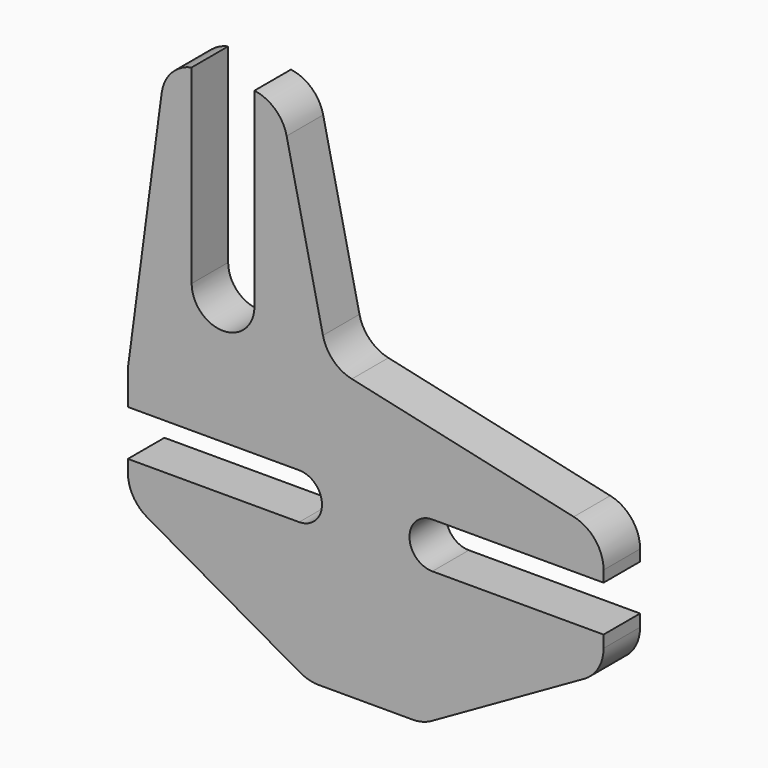
from build123d import *

# Parameters (mm, degrees)
F1_DEPTH     = 12
F2_T1_DEPTH  = 12
F2_T3_DEPTH  = 54.7223945877
F2_T5_DEPTH  = 15.3186487605
F2_T7_DEPTH  = 41.0920435526
F2_T9_DEPTH  = 25.2174840277
F2_T11_DEPTH = 25.2174840277
F2_T13_DEPTH = 41.0920435526
F2_T15_DEPTH = 52.1292425836
F2_T17_DEPTH = 51.6983242764


# Not quite as in the source:
# - a fillet or chamfer that OpenCascade refuses, or shapes differently, is made with other operations: its cross-section is extruded or revolved along the edge and cut away or added


with BuildPart() as f1:
    # F0 (on Front) → F1 (new body)
    with BuildSketch(Plane.XZ):
        with BuildLine():
            Line((-52.5, 90), (-62.5, 15))
            Line((-62.5, 15), (-62.5, 6))
            Line((-62.5, 6), (-17.5, 6))
            ThreePointArc((-17.5, 6), (-11.5, 0), (-17.5, -6))
            Line((-17.5, -6), (-62.5, -6))
            Line((-62.5, -6), (-62.5, -15))
            Line((-62.5, -15), (-15, -42))
            Line((-15, -42), (15, -42))
            Line((15, -42), (62.5, -15))
            Line((62.5, -15), (62.5, -6))
            Line((62.5, -6), (17.5, -6))
            ThreePointArc((17.5, -6), (11.5, 0), (17.5, 6))
            Line((17.5, 6), (62.5, 6))
            Line((62.5, 6), (62.5, 16.9622953511))
            Line((62.5, 16.9622953511), (-9.86454105, 33.0051278665))
            Line((-9.86454105, 33.0051278665), (-22.5, 90))
            Line((-22.5, 90), (-29.25, 90))
            Line((-29.25, 90), (-29.25, 40))
            ThreePointArc((-29.25, 40), (-37.5, 31.75), (-45.75, 40))
            Line((-45.75, 40), (-45.75, 90))
            Line((-45.75, 90), (-52.5, 90))
        make_face()
    extrude(amount=F1_DEPTH)

    # F2: fillet of radius 10 on 9 edges, made by hand

    # F2_s2 → F2_t1 (join)
    with BuildSketch(Plane.XZ):
        with BuildLine():
            ThreePointArc((-3.6448495312, 31.6262554535), (-8.5515212037, 34.3181477128), (-11.243413463, 39.2248193853))
            Line((-11.243413463, 39.2248193853), (-9.86454105, 33.0051278665))
            Line((-9.86454105, 33.0051278665), (-3.6448495312, 31.6262554535))
        make_face()
    extrude(amount=F2_T1_DEPTH)

    # F2_s4 → F2_t3 (cut)
    with BuildSketch(Plane.XZ.offset(-21.3611972939)):
        with BuildLine():
            ThreePointArc((-53.62927012, 81.5304741001), (-51.0385819893, 87.0201735553), (-45.75, 90))
            Line((-45.75, 90), (-52.5, 90))
            Line((-52.5, 90), (-53.62927012, 81.5304741001))
        make_face()
    extrude(amount=F2_T3_DEPTH, mode=Mode.SUBTRACT)

    # F2_s6 → F2_t5 (cut)
    with BuildSketch(Plane.XZ.offset(-1.6593243803)):
        with BuildLine():
            ThreePointArc((-62.4122790068, 15.6579074488), (-62.478045652, 14.9985428246), (-62.5, 14.3362702479))
            Line((-62.5, 14.3362702479), (-62.5, 15))
            Line((-62.5, 15), (-62.4122790068, 15.6579074488))
        make_face()
    extrude(amount=F2_T5_DEPTH, mode=Mode.SUBTRACT)

    # F2_s8 → F2_t7 (cut)
    with BuildSketch(Plane.XZ.offset(-14.5460217763)):
        with BuildLine():
            ThreePointArc((-57.4416662495, -17.875263395), (-61.1433981308, -14.2106735867), (-62.5, -9.1815912895))
            Line((-62.5, -9.1815912895), (-62.5, -15))
            Line((-62.5, -15), (-57.4416662495, -17.875263395))
        make_face()
    extrude(amount=F2_T7_DEPTH, mode=Mode.SUBTRACT)

    # F2_s10 → F2_t9 (cut)
    with BuildSketch(Plane.XZ.offset(-6.6087420138)):
        with BuildLine():
            ThreePointArc((-12.3565031945, -42), (-14.9122104297, -41.6679036263), (-17.2981694439, -40.6936721056))
            Line((-17.2981694439, -40.6936721056), (-15, -42))
            Line((-15, -42), (-12.3565031945, -42))
        make_face()
    extrude(amount=F2_T9_DEPTH, mode=Mode.SUBTRACT)

    # F2_s12 → F2_t11 (cut)
    with BuildSketch(Plane.XZ.offset(-6.6087420138)):
        with BuildLine():
            ThreePointArc((17.2981694439, -40.6936721056), (14.9122104297, -41.6679036263), (12.3565031945, -42))
            Line((12.3565031945, -42), (15, -42))
            Line((15, -42), (17.2981694439, -40.6936721056))
        make_face()
    extrude(amount=F2_T11_DEPTH, mode=Mode.SUBTRACT)

    # F2_s14 → F2_t13 (cut)
    with BuildSketch(Plane.XZ.offset(-14.5460217763)):
        with BuildLine():
            ThreePointArc((62.5, -9.1815912895), (61.1433981308, -14.2106735867), (57.4416662495, -17.875263395))
            Line((57.4416662495, -17.875263395), (62.5, -15))
            Line((62.5, -15), (62.5, -9.1815912895))
        make_face()
    extrude(amount=F2_T13_DEPTH, mode=Mode.SUBTRACT)

    # F2_s16 → F2_t15 (cut)
    with BuildSketch(Plane.XZ.offset(-20.0646212918)):
        with BuildLine():
            ThreePointArc((54.6643961394, 18.6994069056), (60.2988448309, 15.1956815563), (62.5, 8.9364468344))
            Line((62.5, 8.9364468344), (62.5, 16.9622953511))
            Line((62.5, 16.9622953511), (54.6643961394, 18.6994069056))
        make_face()
    extrude(amount=F2_T15_DEPTH, mode=Mode.SUBTRACT)

    # F2_s18 → F2_t17 (cut)
    with BuildSketch(Plane.XZ.offset(-19.8491621382)):
        with BuildLine():
            ThreePointArc((-29.25, 90), (-23.7926014307, 87.4605787727), (-20.7815420039, 82.2485369039))
            Line((-20.7815420039, 82.2485369039), (-22.5, 90))
            Line((-22.5, 90), (-29.25, 90))
        make_face()
    extrude(amount=F2_T17_DEPTH, mode=Mode.SUBTRACT)


solid = f1.part
